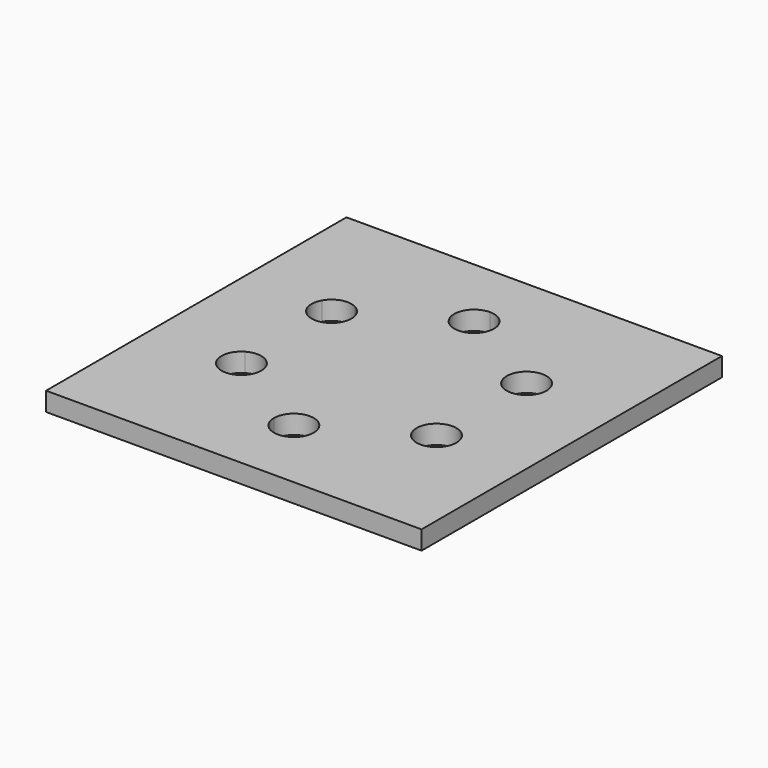
from build123d import *

# Parameters (mm, degrees)
F0_W            = 100
F0_H            = 100
F1_DEPTH        = 5
F3_DEPTH        = 25
F3_COPIES_COUNT = 6


# Not quite as in the source:
# - a pattern or mirror of a feature is missing from the dataset's text; its kind, count and spacing are read off the source's solid


with BuildPart() as f1:
    # F0 (on Top) → F1 (new body)
    with BuildSketch(Plane.XY):
        with Locations((50, 50)):
            Rectangle(F0_W, F0_H)
    extrude(amount=F1_DEPTH)

    # F2 (on face) → F3 (cut)
    with BuildSketch(Plane.XY.offset(5)):
        with BuildLine():
            ThreePointArc((50, 85.3), (46.2523340597, 76.2523340597), (55.3, 80))
            ThreePointArc((55.3, 80), (53.7476659403, 83.7476659403), (50, 85.3))
        make_face()
    f3 = extrude(amount=-F3_DEPTH, mode=Mode.SUBTRACT)

    # F3_copies: F3 ×6 about axis
    f3_copies_axis = Axis((50, 50, 0), (0, 0, 1))
    for i in range(1, F3_COPIES_COUNT):
        add(f3.rotate(f3_copies_axis, i * 360 / F3_COPIES_COUNT), mode=Mode.SUBTRACT)


solid = f1.part
